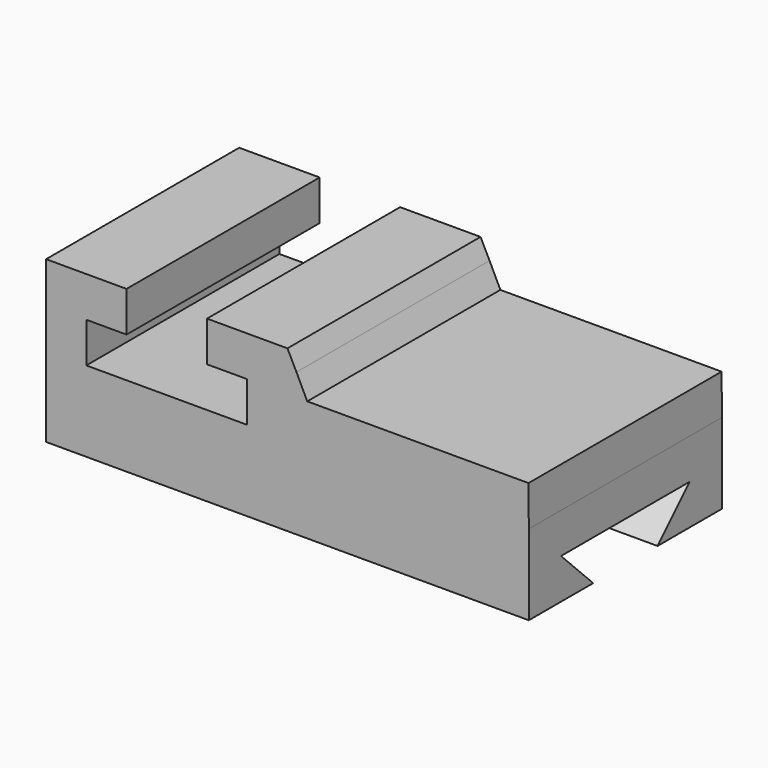
from build123d import *

# Parameters (mm, degrees)
F1_DEPTH = 76.2
F3_DEPTH = 152.4


# Not quite as in the source:
# - a feature names something its author has since deleted; it is built from what else it names


with BuildPart() as f1:
    # F0 (on Front) → F1 (new body)
    with BuildSketch(Plane.XZ):
        Polygon((-76.2, 25.4), (-76.2, 0), (76.2, 0), (76.2, 25.4), (76.1036425829, 38.1), (6.2536425829, 38.1), (2.8439569287, 45.1241247356), (0, 50.8), (-25.4, 50.8), (-25.4, 38.1), (-12.7, 38.1), (-12.7, 25.4), (-63.5, 25.4), (-63.5, 38.1), (-50.8, 38.1), (-50.8, 50.8), (-76.2, 50.8), align=None)
    extrude(amount=F1_DEPTH)

    # F2 (on face) → F3 (cut)
    with BuildSketch(Plane.YZ.offset(76.2)):
        Polygon((-63.5, 12.7), (-50.8, 0), (-38.1, 0), (-38.1, 12.7), align=None)
        Polygon((-38.1, 12.7), (-38.1, 0), (-25.4, 0), (-12.7, 12.7), align=None)
    extrude(amount=-F3_DEPTH, mode=Mode.SUBTRACT)


solid = f1.part
